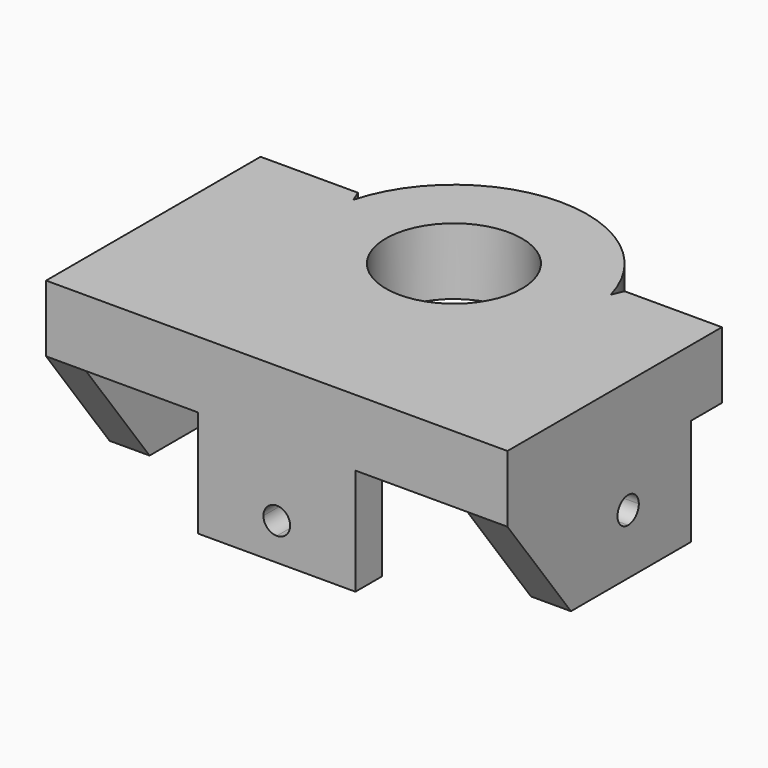
from build123d import *

# Parameters (mm, degrees)
F0_R     = 12.7
F0_R_2   = 6.477
F1_DEPTH = 6.35
F3_DEPTH = 6.35
F5_DEPTH = 3.81
F7_DEPTH = 10.16
F9_DEPTH = 25.4


# Not quite as in the source:
# - a pattern or mirror of a feature is missing from the dataset's text; its kind, count and spacing are read off the source's solid


with BuildPart() as f1:
    # F0 (on Top) → F1 (new body)
    with BuildSketch(Plane.XY):
        Circle(F0_R)
        Circle(F0_R_2, mode=Mode.SUBTRACT)
    extrude(amount=F1_DEPTH)

    # F2 (on face) → F3 (join)
    with BuildSketch(Plane.XY.offset(6.35)):
        Polygon((-21.971, -21.0888834), (0, -21.0888834), (21.971, -21.0888834), (21.971, -17.9138834), (21.971, 4.445), (12.7, 4.445), (6.7730685696, -9.7721947122), (-6.9460314699, -9.7721947122), (-12.7, 4.445), (-21.971, 4.445), (-21.971, -17.907), align=None)
    extrude(amount=-F3_DEPTH)

    # F4 (on face) → F5 (join)
    with BuildSketch(Plane.YZ.offset(21.971)):
        Polygon((0.7805166, 6.35), (-21.0888834, 6.35), (-21.0888834, 0), (-13.5309724137, -10.16), (-6.7194938, -10.16), (0.7805166, -10.16), align=None)
        with BuildLine():
            ThreePointArc((-5.4494938, -4.445), (-5.8214681879, -5.3430256121), (-6.7194938, -5.715))
            ThreePointArc((-6.7194938, -5.715), (-7.6175194121, -3.5469743879), (-5.4494938, -4.445))
        make_face(mode=Mode.SUBTRACT)
    f5 = extrude(amount=-F5_DEPTH)

    # F5_copies: F5 across plane
    add(f5.mirror(Plane(origin=(0, 0, 0), x_dir=(0, 0, -1), z_dir=(-1, 0, 0))))

    # F6 (on face) → F7 (join)
    with BuildSketch(Plane(origin=(0, 0, 0), x_dir=(1, 0, 0), z_dir=(0, 0, -1))):
        Polygon((7.493, 21.0888834), (0, 21.0888834), (-7.493, 21.0888834), (-7.493, 17.9138834), (7.493, 17.9138834), align=None)
    extrude(amount=F7_DEPTH)

    # F8 (on face) → F9 (cut)
    with BuildSketch(Plane(origin=(0, -17.9138834, 0), x_dir=(-1, 0, 0), z_dir=(0, 1, 0))):
        with BuildLine():
            ThreePointArc((0, -7.912179098), (0.8980256121, -7.5402047101), (1.27, -6.642179098))
            ThreePointArc((1.27, -6.642179098), (-0.8980256121, -5.7441534859), (0, -7.912179098))
        make_face()
    extrude(amount=-F9_DEPTH, mode=Mode.SUBTRACT)


solid = f1.part
